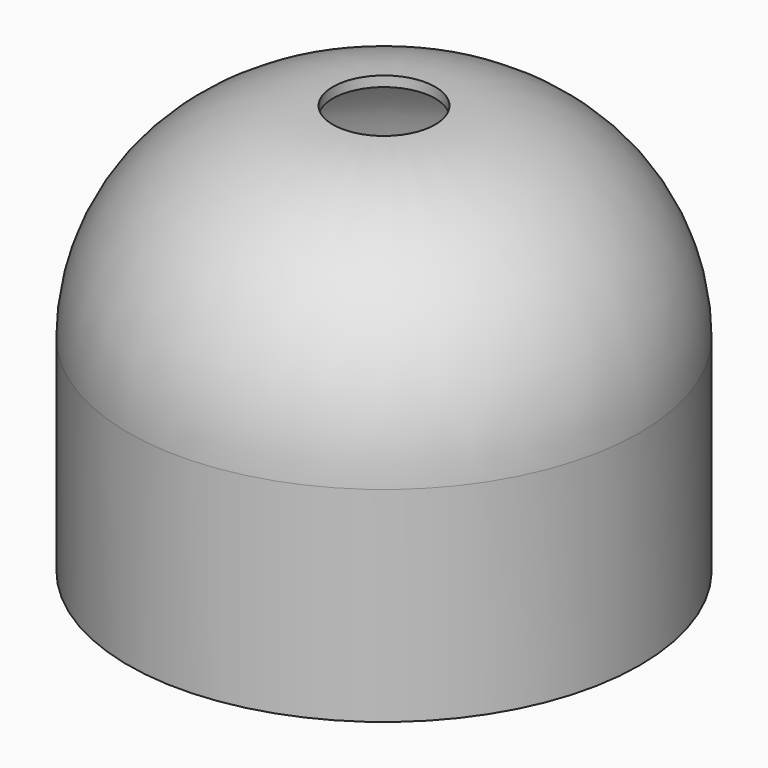
from build123d import *

# Parameters (mm, degrees)
F0_R     = 25
F1_DEPTH = 40
F2_R     = 20
F3_T     = -1


# Not quite as in the source:
# - a fillet or chamfer that OpenCascade refuses, or shapes differently, is made with other operations: its cross-section is extruded or revolved along the edge and cut away or added


with BuildPart() as f1:
    # F0 (on Top) → F1 (new body)
    with BuildSketch(Plane.XY):
        Circle(F0_R)
    extrude(amount=F1_DEPTH)

    # F2
    f2_edges = [f1.edges().sort_by_distance(p)[0] for p in [
        (-25, 0, 40),
    ]]
    fillet(f2_edges, radius=F2_R)

    # F3: a shell. OpenCascade refuses it in one call, so the cavity is built on its own and cut out:
    # the body offset inwards by the wall thickness, plus a prism from it out through each open face.
    f3_core = offset(f1.part, amount=F3_T, mode=Mode.PRIVATE)
    f3_exits = [f3_core.faces().sort_by_distance(p)[0] for p in [
        (0, 0, 39),
        (0, 0, 1),
    ]]
    add(f3_core, mode=Mode.SUBTRACT)
    extrude(f3_exits, amount=-F3_T, mode=Mode.SUBTRACT)

    # F4: fillet of radius 2 on 1 edges, made by hand

    # F4_s1 → F4_t2 (revolve, cut)
    with BuildSketch(Plane.XZ):
        with BuildLine():
            ThreePointArc((25, 0), (24.2679491924, 0.7320508076), (24, 1.7320508076))
            Line((24, 1.7320508076), (24, 0))
            Line((24, 0), (25, 0))
        make_face()
    revolve(axis=Axis((0, 0, 0), (0, 0, -1)), mode=Mode.SUBTRACT)


solid = f1.part
